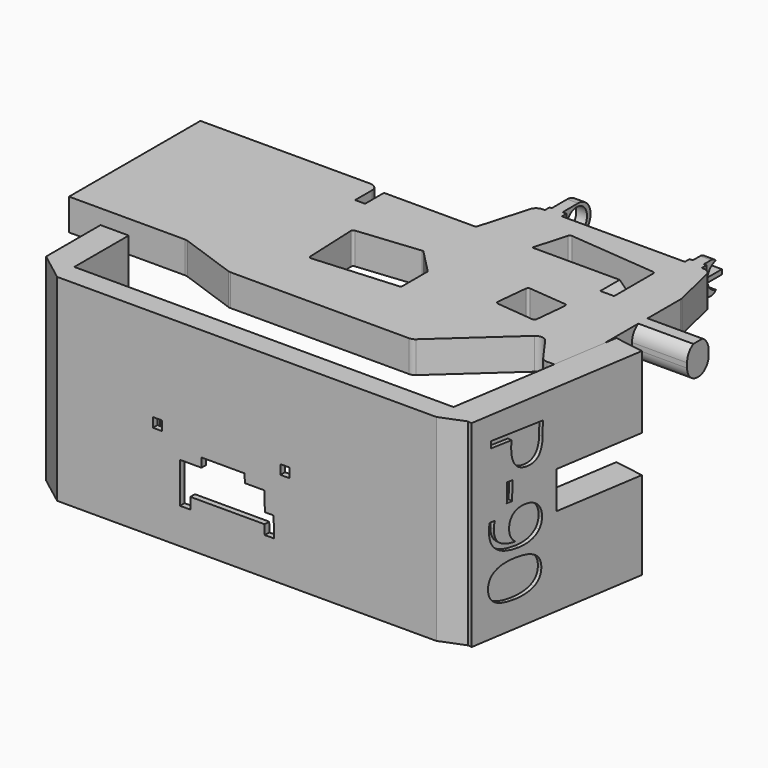
from build123d import *

# Parameters (mm, degrees)
F1_DEPTH     = 4
F3_DEPTH     = 25
F4_R         = 1.7
F5_SIZE      = 1
F7_R         = 1
F9_DEPTH     = 0.5
F10_R        = 0.2
F12_DEPTH    = 25
F13_W        = 4.2640957981
F13_H        = 4.7070300207
F13_W_2      = 7.1971410604
F14_DEPTH    = 4
F16_DEPTH    = 1.4
F17_R        = 1.99999
F18_T1_DEPTH = 5.2538537094
F19_R        = 0.3
F21_DEPTH    = 5
F22_DEPTH    = 2
F24_DEPTH    = 3
F26_DEPTH    = 0.508
F28_DEPTH    = 6.9789886475


# Not quite as in the source:
# - a fillet or chamfer that OpenCascade refuses, or shapes differently, is made with other operations: its cross-section is extruded or revolved along the edge and cut away or added
# - a fillet or chamfer is up to 0.001 mm smaller than in the source, because OpenCascade refuses the exact size


with BuildPart() as f1:
    # F0 (on Top) → F1 (new body)
    with BuildSketch(Plane.XY):
        Polygon((2.6934260968, -5.2742385305), (-19.873496145, -5.2742385305), (-19.8852140456, -26.0831601918), (-4.9857888371, -26.0831601918), (2.5662551634, -28.7642404437), (25.7749762386, -28.7642404437), (35.5768278241, -19.8526754975), (38.6626347899, -24.1568814963), (41.1353074014, -24.1568814963), (41.1353074014, -13.1260063499), (48.1142960489, -13.1260063499), (48.1142960489, -9.7081437707), (41.1497019231, -9.7081437707), (41.1497019231, -5.3435540758), (39.6437942982, 1.0947899427), (38.6000163853, 1.0947899427), (38.6000163853, 1.8441530508), (38.2520891726, 1.8441530508), (38.2520891726, 3.7778269034), (36.8706174195, 3.7778269034), (36.8706174195, 1.8408568576), (36.4612936974, 1.8441530508), (36.4612936974, 1.0947899427), (20.8624477269, 1.0947899427), (20.8624477269, 1.8441530508), (20.3708820045, 1.8408568576), (20.3410126269, 6.2953173183), (18.9800560474, 6.2953173183), (18.9800560474, 1.8365884898), (18.7107231468, 1.8365884898), (18.7107231468, 1.0847063968), (17.6446232945, 1.0847063968), (15.6181209185, -5.9725809842), (14.758749865, -8.965337649), (2.9602518771, -8.965337649), (2.6934260968, -8.965337649), align=None)
        Polygon((6.4800432883, -14.1137875617), (14.7967338562, -13.2744237781), (17.8792309016, -16.4292808622), (17.8792309016, -20.6550508738), (6.798423361, -21.4654710144), align=None, mode=Mode.SUBTRACT)
        Polygon((27.3169986904, -17.448535189), (27.7794320136, -12.9215558991), (33.1285022632, -13.4127461622), (32.6604864311, -17.9943752814), align=None, mode=Mode.SUBTRACT)
        Polygon((21.8643173575, -9.025641717), (22.7453019361, -5.9576160274), (24.017155533, -1.5283903593), (35.5836041272, -2.5712102652), (35.5836041272, -9.025641717), (34.8310694098, -9.025641717), align=None, mode=Mode.SUBTRACT)
        Polygon((2.9602518771, -5.9725809842), (2.9602518771, -8.965337649), (14.758749865, -8.965337649), (15.6181209185, -5.9725809842), align=None)
        Polygon((34.8310694098, -5.9576160274), (22.7453019361, -5.9576160274), (21.8643173575, -9.025641717), (34.8310694098, -9.025641717), align=None)
    extrude(amount=F1_DEPTH)

    # F2 (on face) → F3 (cut)
    with BuildSketch(Plane(origin=(18.9800560474, 0, 0), x_dir=(0, -1, 0), z_dir=(-1, 0, 0))):
        with BuildLine():
            ThreePointArc((-5.2999777311, 3.1070642549), (-5.723785386, 2), (-5.2999777311, 0.8929357451))
            Line((-5.2999777311, 0.8929357451), (-4.0659529041, 2))
            Line((-4.0659529041, 2), (-5.2999777311, 3.1070642549))
        make_face()
        with BuildLine():
            Line((-4.0659529041, 2), (-5.2999777311, 0.8929357451))
            ThreePointArc((-5.2999777311, 0.8929357451), (-4.0659529041, 0.342167518), (-2.831928077, 0.8929357451))
            Line((-2.831928077, 0.8929357451), (-4.0659529041, 2))
        make_face()
        with BuildLine():
            Line((-5.2999777311, 3.1070642549), (-4.0659529041, 2))
            Line((-4.0659529041, 2), (-2.831928077, 3.1070642549))
            ThreePointArc((-2.831928077, 3.1070642549), (-4.0659529041, 3.657832482), (-5.2999777311, 3.1070642549))
        make_face()
        with BuildLine():
            Line((-2.831928077, 3.1070642549), (-4.0659529041, 2))
            Line((-4.0659529041, 2), (-2.831928077, 0.8929357451))
            ThreePointArc((-2.831928077, 0.8929357451), (-2.5176934006, 1.4072934552), (-2.4081204221, 2))
            ThreePointArc((-2.4081204221, 2), (-2.5176934006, 2.5927065448), (-2.831928077, 3.1070642549))
        make_face()
    extrude(amount=-F3_DEPTH, mode=Mode.SUBTRACT)

    # F4
    f4_edges = [f1.edges().sort_by_distance(p)[0] for p in [
        (44.631999, -9.708144, 4),
        (44.631999, -9.708144, 0),
        (44.624802, -13.126006, 4),
        (44.624802, -13.126006, 0),
    ]]
    fillet(f4_edges, radius=F4_R)

    # F5
    f5_edges = [f1.edges().sort_by_distance(p)[0] for p in [
        (2.960252, -7.468959, 4),
        (2.960252, -7.468959, 0),
        (34.831069, -7.491629, 4),
        (34.831069, -7.491629, 0),
    ]]
    chamfer(f5_edges, length=F5_SIZE)

    # F7
    f7_edges = [f1.edges().sort_by_distance(p)[0] for p in [
        (-4.985789, -26.08316, 2),
        (2.566255, -28.76424, 2),
        (25.774976, -28.76424, 2),
        (35.576828, -19.852675, 2),
        (38.662635, -24.156881, 2),
        (41.135307, -24.156881, 2),
        (41.149702, -5.343554, 2),
        (39.643794, 1.09479, 2),
        (17.644623, 1.084706, 2),
        (2.693426, -5.274239, 2),
    ]]
    fillet(f7_edges, radius=F7_R)

    # F8 (on face) → F9 (join)
    with BuildSketch(Plane(origin=(0, -5.9725809842, 0), x_dir=(-1, 0, 0), z_dir=(0, 1, 0))):
        Polygon((-4.663484171, 0.6533203996), (-4.2501688004, 0.6387769245), (-4.2501688004, 3.2442298252), (-4.663484171, 3.2442298252), align=None)
        Polygon((-7, 0.6), (-6.5866846293, 0.5854565249), (-6.5866846293, 3.1909094256), (-7, 3.1909094256), align=None)
        Polygon((-9.336515829, 0.5466796004), (-8.9232004583, 0.5321361253), (-8.9232004583, 3.1375890261), (-9.336515829, 3.1375890261), align=None)
        Polygon((-11.6730316579, 0.4933592008), (-11.2597162873, 0.4788157257), (-11.2597162873, 3.0842686265), (-11.6730316579, 3.0842686265), align=None)
        Polygon((-14.0095474869, 0.4400388013), (-13.5962321162, 0.4254953261), (-13.5962321162, 3.0309482269), (-14.0095474869, 3.0309482269), align=None)
        Polygon((-16.3460633159, 0.3867184017), (-15.9327479452, 0.3721749266), (-15.9327479452, 2.9776278273), (-16.3460633159, 2.9776278273), align=None)
        Polygon((-18.6825791448, 0.3333980021), (-18.2692637742, 0.318854527), (-18.2692637742, 2.9243074277), (-18.6825791448, 2.9243074277), align=None)
        Polygon((-21.0190949738, 0.2800776025), (-20.6057796031, 0.2655341274), (-20.6057796031, 2.8709870282), (-21.0190949738, 2.8709870282), align=None)
        Polygon((-23.3556108028, 0.2267572029), (-22.9422954321, 0.2122137278), (-22.9422954321, 2.8176666286), (-23.3556108028, 2.8176666286), align=None)
        Polygon((-25.6921266317, 0.1734368034), (-25.2788112611, 0.1588933283), (-25.2788112611, 2.764346229), (-25.6921266317, 2.764346229), align=None)
        Polygon((-28.0286424607, 0.1201164038), (-27.61532709, 0.1055729287), (-27.61532709, 2.7110258294), (-28.0286424607, 2.7110258294), align=None)
        Polygon((-30.3651582897, 0.0667960042), (-29.951842919, 0.0522525291), (-29.951842919, 2.6577054298), (-30.3651582897, 2.6577054298), align=None)
        Polygon((-32.7016741186, 0.0134756046), (-32.288358748, -0.0010678705), (-32.288358748, 2.6043850303), (-32.7016741186, 2.6043850303), align=None)
    extrude(amount=F9_DEPTH)

    # F10
    f10_edges = [f1.edges().sort_by_distance(p)[0] for p in [
        (4.250169, -5.472581, 1.941503),
        (4.663484, -5.472581, 1.948775),
        (6.586685, -5.472581, 1.888183),
        (7, -5.472581, 1.895455),
        (8.9232, -5.472581, 1.834863),
        (9.336516, -5.472581, 1.842134),
        (11.259716, -5.472581, 1.781542),
        (11.673032, -5.472581, 1.788814),
        (13.596232, -5.472581, 1.728222),
        (14.009547, -5.472581, 1.735494),
        (23.355611, -5.472581, 1.522212),
        (22.942295, -5.472581, 1.51494),
        (25.692127, -5.472581, 1.468892),
        (25.278811, -5.472581, 1.46162),
        (27.615327, -5.472581, 1.408299),
        (28.028642, -5.472581, 1.415571),
        (29.951843, -5.472581, 1.354979),
        (30.365158, -5.472581, 1.362251),
        (32.288359, -5.472581, 1.301659),
        (32.701674, -5.472581, 1.30893),
    ]]
    fillet(f10_edges, radius=F10_R)

    # F15 (on face) → F16 (join)
    with BuildSketch(Plane(origin=(36.8706174195, 0, 0), x_dir=(0, -1, 0), z_dir=(-1, 0, 0))):
        with BuildLine():
            ThreePointArc((-2.4346986369, 1.7043345571), (-2.414778345, 1.8515711823), (-2.4081204221, 2))
            Line((-2.4081204221, 2), (-4.7012325376, 2))
            Line((-4.7012325376, 2), (-4.7012325376, 1.7043345571))
            Line((-4.7012325376, 1.7043345571), (-2.4346986369, 1.7043345571))
        make_face()
        with BuildLine():
            Line((-4.7012325376, 2), (-2.4081204221, 2))
            ThreePointArc((-2.4081204221, 2), (-2.414778345, 2.1484288177), (-2.4346986369, 2.2956654429))
            Line((-2.4346986369, 2.2956654429), (-4.7012325376, 2.2956654429))
            Line((-4.7012325376, 2.2956654429), (-4.7012325376, 2))
        make_face()
    extrude(amount=-F16_DEPTH)

    # F17 (radius 2 in the source; OpenCascade refuses exactly that, so slightly less here)
    f17_edges = [f1.edges().sort_by_distance(p)[0] for p in [
        (19.660534, 6.295317, 0),
        (19.660534, 6.295317, 4),
    ]]
    fillet(f17_edges, radius=F17_R)

    # F18: fillet of radius 1 on 2 edges, made by hand

    # F18_s2 → F18_t1 (cut)
    with BuildSketch(Plane.YZ.offset(34.9344264413)):
        with BuildLine():
            ThreePointArc((3.0033505121, 4), (3.431951251, 3.9034939992), (3.7778269034, 3.6326028133))
            Line((3.7778269034, 3.6326028133), (3.7778269034, 4))
            Line((3.7778269034, 4), (3.0033505121, 4))
        make_face()
        with BuildLine():
            ThreePointArc((3.0033505121, 0), (3.431951251, 0.0965060008), (3.7778269034, 0.3673971867))
            Line((3.7778269034, 0.3673971867), (3.7778269034, 0))
            Line((3.7778269034, 0), (3.0033505121, 0))
        make_face()
    extrude(amount=F18_T1_DEPTH, mode=Mode.SUBTRACT)

    # F19
    f19_edges = [f1.edges().sort_by_distance(p)[0] for p in [
        (24.017156, -1.52839, 2),
        (35.583604, -2.57121, 2),
        (33.128502, -13.412746, 2),
        (32.660486, -17.994375, 2),
        (27.316999, -17.448535, 2),
        (27.779432, -12.921556, 2),
        (17.879231, -16.429281, 2),
        (17.879231, -20.655051, 2),
        (14.796734, -13.274424, 2),
        (6.480043, -14.113788, 2),
        (6.798423, -21.465471, 2),
    ]]
    fillet(f19_edges, radius=F19_R)

    # F27 (on face) → F28 (join, through all)
    with BuildSketch(Plane.YZ.offset(48.1142960489)):
        with BuildLine():
            Line((-9.7081437707, 2.3), (-13.1260063499, 2.3))
            Line((-13.1260063499, 2.3), (-13.1260063499, 1.7))
            ThreePointArc((-13.1260063499, 1.7), (-12.6280878779, 0.497918472), (-11.4260063499, 0))
            Line((-11.4260063499, 0), (-11.4081437707, 0))
            ThreePointArc((-11.4081437707, 0), (-10.2060622427, 0.497918472), (-9.7081437707, 1.7))
            Line((-9.7081437707, 1.7), (-9.7081437707, 2.3))
        make_face()
        with BuildLine():
            Line((-11.4081437707, 4), (-11.4260063499, 4))
            ThreePointArc((-11.4260063499, 4), (-12.6280878779, 3.502081528), (-13.1260063499, 2.3))
            Line((-13.1260063499, 2.3), (-9.7081437707, 2.3))
            ThreePointArc((-9.7081437707, 2.3), (-10.2060622427, 3.502081528), (-11.4081437707, 4))
        make_face()
        with BuildLine():
            ThreePointArc((-13.1260063499, 2.3), (-12.6280878779, 3.502081528), (-11.4260063499, 4))
            Line((-11.4260063499, 4), (-12.1334744617, 4))
            ThreePointArc((-12.1334744617, 4), (-12.8597103306, 3.2842661669), (-13.1260063499, 2.3))
        make_face()
        with BuildLine():
            Line((-10.6828130797, 4), (-11.4081437707, 4))
            ThreePointArc((-11.4081437707, 4), (-10.2060622427, 3.502081528), (-9.7081437707, 2.3))
            ThreePointArc((-9.7081437707, 2.3), (-9.9667172587, 3.2811567577), (-10.6828130797, 4))
        make_face()
    extrude(amount=-F28_DEPTH)


with BuildPart() as f12:
    # F11 (on face) → F12 (new body)
    with BuildSketch(Plane.XY.offset(4)):
        Polygon((44.5833335705, -16.4324613858), (41.3761623204, -15.9014053643), (38.0217470229, -37.5300385058), (-10.0583480671, -37.5300385058), (-10.0583480671, -28.9046149701), (-13.636412099, -28.9046149701), (-13.636412099, -37.5300385058), (-10.0583480671, -40.2552820742), (38.0217470229, -40.2552820742), (41.0766750574, -39.0427298844), align=None)
    extrude(amount=-F12_DEPTH)

    # F13 (on face) → F14 (cut)
    with BuildSketch(Plane(origin=(46.0248163774, -7.1380538526, 0), x_dir=(0.1532591685, 0.9881860287, 0), z_dir=(0.9881860287, -0.1532591685, 0))):
        Polygon((-7.2025824338, -5.1408624277), (-9.4055241255, -5.1408624277), (-16.6026651859, -5.1408624277), (-16.6026651859, -9.8478924483), (-9.4055241255, -9.8478924483), (-7.2025824338, -10.2310068905), align=None)
        with Locations((-18.734713085, -7.494377438)):
            Rectangle(F13_W, F13_H)
        with Locations((-13.0040946557, -7.494377438)):
            Rectangle(F13_W_2, F13_H)
    extrude(amount=-F14_DEPTH, mode=Mode.SUBTRACT)

    # F20 (on face) → F21 (cut)
    with BuildSketch(Plane(origin=(0, -37.5300385058, 0), x_dir=(-1, 0, 0), z_dir=(0, 1, 0))):
        Polygon((-10.7441206637, -15.0589602471), (-10.7441206637, -10.204165907), (-13.7182893232, -10.204165907), (-13.74556683, -11.2833930179), (-16.2131562829, -11.2833930179), (-16.2884704769, -13.7014463544), (-17.4019206315, -13.7014463544), (-17.4291040748, -16.2507686764), (-16.2706725371, -16.2631210407), (-16.2578325614, -15.0589602471), align=None)
        Polygon((-8.2328791401, -10.204165907), (-10.7441206637, -10.204165907), (-10.7441206637, -15.0589602471), (-6.8352012895, -15.0589602471), (-6.8352012895, -16.4881702513), (-5.5278930813, -16.4881702513), (-5.5278930813, -11.3542200997), (-8.2451421767, -11.3542200997), align=None)
        Polygon((-18.2534381747, -7.6958201826), (-19.4096304476, -7.6958201826), (-19.4027870893, -8.8917091489), (-18.2534381747, -8.8917091489), align=None)
        Polygon((-2.0786108798, -7.6958201826), (-3.2348031527, -7.6958201826), (-3.2348031527, -8.8917091489), (-2.0854542381, -8.8917091489), align=None)
    extrude(amount=-F21_DEPTH, mode=Mode.SUBTRACT)

    # F20 (on face) → F22 (cut)
    with BuildSketch(Plane(origin=(0, -37.5300385058, 0), x_dir=(-1, 0, 0), z_dir=(0, 1, 0))):
        Polygon((-0.7839830942, 1.2256489135), (-10.7441206637, 1.2256489135), (-10.7441206637, -10.204165907), (-8.2328791401, -10.204165907), (-8.2451421767, -11.3542200997), (-5.5278930813, -11.3542200997), (-5.5278930813, -16.4881702513), (-6.8352012895, -16.4881702513), (-6.8352012895, -15.0589602471), (-10.7441206637, -15.0589602471), (-10.7441206637, -18.6946262256), (-0.7839830942, -18.6946262256), align=None)
        Polygon((-3.2348031527, -8.8917091489), (-3.2348031527, -7.6958201826), (-2.0786108798, -7.6958201826), (-2.0854542381, -8.8917091489), align=None, mode=Mode.SUBTRACT)
        Polygon((-10.7441206637, 1.2256489135), (-20.7042582333, 1.2256489135), (-20.7042582333, -18.6946262256), (-10.7441206637, -18.6946262256), (-10.7441206637, -15.0589602471), (-16.2578325614, -15.0589602471), (-16.2706725371, -16.2631210407), (-17.4291040748, -16.2507686764), (-17.4019206315, -13.7014463544), (-16.2884704769, -13.7014463544), (-16.2131562829, -11.2833930179), (-13.74556683, -11.2833930179), (-13.7182893232, -10.204165907), (-10.7441206637, -10.204165907), align=None)
        Polygon((-19.4027870893, -8.8917091489), (-19.4096304476, -7.6958201826), (-18.2534381747, -7.6958201826), (-18.2534381747, -8.8917091489), align=None, mode=Mode.SUBTRACT)
    extrude(amount=-F22_DEPTH, mode=Mode.SUBTRACT)

    # F23 (on face) → F24 (cut)
    with BuildSketch(Plane(origin=(-13.636412099, 0, 0), x_dir=(0, -1, 0), z_dir=(-1, 0, 0))):
        with BuildLine():
            Line((35.6485965423, -20.3161685267), (33.5925474496, -20.1962334233))
            Line((33.5925474496, -20.1962334233), (33.6680283577, -20.6826224671))
            Line((33.6680283577, -20.6826224671), (35.6674124532, -20.800094644))
            add(Edge.make_bspline(
                [(36.170021659, -20.7868217916), (35.9923202004, -20.8143986206), (35.6674124532, -20.800094644)],
                knots=[0, 0, 0, 1, 1, 1], degree=2))
            add(Edge.make_bspline(
                [(36.7059816488, -20.4897735703), (36.5391643796, -20.7295359047), (36.170021659, -20.7868217916)],
                knots=[0, 0, 0, 1, 1, 1], degree=2))
            add(Edge.make_bspline(
                [(36.8159394769, -19.8836164761), (36.8727989181, -20.250011236), (36.7059816488, -20.4897735703)],
                knots=[0, 0, 0, 1, 1, 1], degree=2))
            add(Edge.make_bspline(
                [(36.5935289668, -19.3782858258), (36.7737213418, -19.6115683668), (36.8159394769, -19.8836164761)],
                knots=[0, 0, 0, 1, 1, 1], degree=2))
            add(Edge.make_bspline(
                [(36.0126042282, -18.9201492485), (36.4133365917, -19.1450032847), (36.5935289668, -19.3782858258)],
                knots=[0, 0, 0, 1, 1, 1], degree=2))
            Line((36.0126042282, -18.9201492485), (36.0073447299, -18.8862577332))
            Line((36.0073447299, -18.8862577332), (36.5977465295, -18.8584226281))
            Line((36.5977465295, -18.8584226281), (36.5360540358, -18.4608843136))
            Line((36.5360540358, -18.4608843136), (33.2961676124, -18.286400737))
            Line((33.2961676124, -18.286400737), (33.3699427373, -18.7617979381))
            Line((33.3699427373, -18.7617979381), (34.7736176608, -18.836637324))
            add(Edge.make_bspline(
                [(35.5907766713, -19.0006198421), (35.2413250899, -18.8644265124), (34.7736176608, -18.836637324)],
                knots=[0, 0, 0, 1, 1, 1], degree=2))
            add(Edge.make_bspline(
                [(36.1497162504, -19.3533548306), (35.9402282526, -19.1368131717), (35.5907766713, -19.0006198421)],
                knots=[0, 0, 0, 1, 1, 1], degree=2))
            add(Edge.make_bspline(
                [(36.3982951141, -19.8217928869), (36.3592042482, -19.5698964894), (36.1497162504, -19.3533548306)],
                knots=[0, 0, 0, 1, 1, 1], degree=2))
            add(Edge.make_bspline(
                [(36.0542373272, -20.3066872863), (36.4636834714, -20.2431468608), (36.3982951141, -19.8217928869)],
                knots=[0, 0, 0, 1, 1, 1], degree=2))
            add(Edge.make_bspline(
                [(35.6485965423, -20.3161685267), (35.9113433708, -20.3288624684), (36.0542373272, -20.3066872863)],
                knots=[0, 0, 0, 1, 1, 1], degree=2))
        make_face()
        with BuildLine():
            Line((34.0340840387, -15.4130917276), (36.0811785063, -15.529726234))
            Line((36.0811785063, -15.529726234), (36.0056975981, -15.0433371902))
            Line((36.0056975981, -15.0433371902), (34.0185846828, -14.9324031122))
            add(Edge.make_bspline(
                [(33.4926493588, -14.9464817188), (33.7188981231, -14.9113710139), (34.0185846828, -14.9324031122)],
                knots=[0, 0, 0, 1, 1, 1], degree=2))
            add(Edge.make_bspline(
                [(32.9688104215, -15.2430559887), (33.1354144678, -15.001919674), (33.4926493588, -14.9464817188)],
                knots=[0, 0, 0, 1, 1, 1], degree=2))
            add(Edge.make_bspline(
                [(32.8586393705, -15.8478391026), (32.8022063752, -15.4841923033), (32.9688104215, -15.2430559887)],
                knots=[0, 0, 0, 1, 1, 1], degree=2))
            add(Edge.make_bspline(
                [(33.0857404161, -16.3561940318), (32.9012839514, -16.1226351725), (32.8586393705, -15.8478391026)],
                knots=[0, 0, 0, 1, 1, 1], degree=2))
            add(Edge.make_bspline(
                [(33.6618324706, -16.8103903433), (33.2701968808, -16.589752891), (33.0857404161, -16.3561940318)],
                knots=[0, 0, 0, 1, 1, 1], degree=2))
            Line((33.6618324706, -16.8103903433), (33.6663812259, -16.839701924))
            Line((33.6663812259, -16.839701924), (33.0758372778, -16.8666210422))
            Line((33.0758372778, -16.8666210422), (33.1375297715, -17.2641593568))
            Line((33.1375297715, -17.2641593568), (36.3788376809, -17.4478028023))
            Line((36.3788376809, -17.4478028023), (36.3042096643, -16.9669096799))
            Line((36.3042096643, -16.9669096799), (34.8999661464, -16.8884063463))
            add(Edge.make_bspline(
                [(34.086336914, -16.7290353104), (34.4328273117, -16.8642811055), (34.8999661464, -16.8884063463)],
                knots=[0, 0, 0, 1, 1, 1], degree=2))
            add(Edge.make_bspline(
                [(33.5305717413, -16.3786218368), (33.7398465162, -16.5937895153), (34.086336914, -16.7290353104)],
                knots=[0, 0, 0, 1, 1, 1], degree=2))
            add(Edge.make_bspline(
                [(33.2816375062, -15.9078938132), (33.3212969664, -16.1634541583), (33.5305717413, -16.3786218368)],
                knots=[0, 0, 0, 1, 1, 1], degree=2))
            add(Edge.make_bspline(
                [(33.3403193418, -15.5667187669), (33.2470953957, -15.6853089966), (33.2816375062, -15.9078938132)],
                knots=[0, 0, 0, 1, 1, 1], degree=2))
            add(Edge.make_bspline(
                [(33.6130767203, -15.4202674111), (33.433543288, -15.4481285373), (33.3403193418, -15.5667187669)],
                knots=[0, 0, 0, 1, 1, 1], degree=2))
            add(Edge.make_bspline(
                [(34.0340840387, -15.4130917276), (33.7275750828, -15.4024988357), (33.6130767203, -15.4202674111)],
                knots=[0, 0, 0, 1, 1, 1], degree=2))
        make_face()
        with BuildLine():
            add(Edge.make_bspline(
                [(35.369233503, -13.154387338), (35.3447839433, -12.9968375912), (35.2310716928, -12.7537072699)],
                knots=[0, 0, 0, 1, 1, 1], degree=2))
            add(Edge.make_bspline(
                [(35.3194812501, -13.3989649246), (35.3922615767, -13.3027772158), (35.369233503, -13.154387338)],
                knots=[0, 0, 0, 1, 1, 1], degree=2))
            add(Edge.make_bspline(
                [(35.0864032161, -13.520028639), (35.2467009236, -13.4951526334), (35.3194812501, -13.3989649246)],
                knots=[0, 0, 0, 1, 1, 1], degree=2))
            add(Edge.make_bspline(
                [(34.7001403047, -13.5274407456), (34.9572490632, -13.540071592), (35.0864032161, -13.520028639)],
                knots=[0, 0, 0, 1, 1, 1], degree=2))
            Line((34.7001403047, -13.5274407456), (32.9143871376, -13.4265324387))
            Line((32.9143871376, -13.4265324387), (32.7931343793, -12.6451956132))
            Line((32.7931343793, -12.6451956132), (32.4179735432, -12.6274336696))
            Line((32.4179735432, -12.6274336696), (32.5396527474, -13.4115184559))
            Line((32.5396527474, -13.4115184559), (31.7934055106, -13.3659818083))
            Line((31.7934055106, -13.3659818083), (31.8369029831, -13.6462737997))
            Line((31.8369029831, -13.6462737997), (32.5455817464, -13.9030727236))
            Line((32.5455817464, -13.9030727236), (32.8512444425, -14.3978288926))
            Line((32.8512444425, -14.3978288926), (33.0663439942, -14.4057224347))
            Line((33.0663439942, -14.4057224347), (32.9898680458, -13.9129214826))
            Line((32.9898680458, -13.9129214826), (34.7692723998, -14.0091867596))
            add(Edge.make_bspline(
                [(35.2068305777, -13.9938143312), (35.0181372763, -14.0230969434), (34.7692723998, -14.0091867596)],
                knots=[0, 0, 0, 1, 1, 1], degree=2))
            add(Edge.make_bspline(
                [(35.685707472, -13.7248545749), (35.5448297437, -13.9413614967), (35.2068305777, -13.9938143312)],
                knots=[0, 0, 0, 1, 1, 1], degree=2))
            add(Edge.make_bspline(
                [(35.7710050965, -13.1501967751), (35.8265852002, -13.508347653), (35.685707472, -13.7248545749)],
                knots=[0, 0, 0, 1, 1, 1], degree=2))
            add(Edge.make_bspline(
                [(35.7066143584, -12.9256777312), (35.7576431278, -13.0640940066), (35.7710050965, -13.1501967751)],
                knots=[0, 0, 0, 1, 1, 1], degree=2))
            add(Edge.make_bspline(
                [(35.6002144135, -12.6964213829), (35.655585589, -12.7872614558), (35.7066143584, -12.9256777312)],
                knots=[0, 0, 0, 1, 1, 1], degree=2))
            Line((35.6002144135, -12.6964213829), (35.2310716928, -12.7537072699))
        make_face()
        with BuildLine():
            Line((34.3034443124, -11.6481844933), (32.2473952196, -11.5282493898))
            Line((32.2473952196, -11.5282493898), (32.3228761278, -12.0146384336))
            Line((32.3228761278, -12.0146384336), (34.3222602233, -12.1321106105))
            add(Edge.make_bspline(
                [(34.824869429, -12.1188377582), (34.6471679705, -12.1464145872), (34.3222602233, -12.1321106105)],
                knots=[0, 0, 0, 1, 1, 1], degree=2))
            add(Edge.make_bspline(
                [(35.3608294189, -11.8217895369), (35.1940121497, -12.0615518712), (34.824869429, -12.1188377582)],
                knots=[0, 0, 0, 1, 1, 1], degree=2))
            add(Edge.make_bspline(
                [(35.470787247, -11.2156324426), (35.5276466882, -11.5820272026), (35.3608294189, -11.8217895369)],
                knots=[0, 0, 0, 1, 1, 1], degree=2))
            add(Edge.make_bspline(
                [(35.2483767368, -10.7103017923), (35.4285691119, -10.9435843334), (35.470787247, -11.2156324426)],
                knots=[0, 0, 0, 1, 1, 1], degree=2))
            add(Edge.make_bspline(
                [(34.6674519983, -10.252165215), (35.0681843618, -10.4770192512), (35.2483767368, -10.7103017923)],
                knots=[0, 0, 0, 1, 1, 1], degree=2))
            Line((34.6674519983, -10.252165215), (34.6621925, -10.2182736997))
            Line((34.6621925, -10.2182736997), (35.2525942995, -10.1904385947))
            Line((35.2525942995, -10.1904385947), (35.1909018058, -9.7929002801))
            Line((35.1909018058, -9.7929002801), (31.9510153825, -9.6184167036))
            Line((31.9510153825, -9.6184167036), (32.0247905074, -10.0938139046))
            Line((32.0247905074, -10.0938139046), (33.4284654309, -10.1686532906))
            add(Edge.make_bspline(
                [(34.2456244413, -10.3326358086), (33.89617286, -10.196442479), (33.4284654309, -10.1686532906)],
                knots=[0, 0, 0, 1, 1, 1], degree=2))
            add(Edge.make_bspline(
                [(34.8045640205, -10.6853707971), (34.5950760227, -10.4688291382), (34.2456244413, -10.3326358086)],
                knots=[0, 0, 0, 1, 1, 1], degree=2))
            add(Edge.make_bspline(
                [(35.0531428841, -11.1538088534), (35.0140520183, -10.901912456), (34.8045640205, -10.6853707971)],
                knots=[0, 0, 0, 1, 1, 1], degree=2))
            add(Edge.make_bspline(
                [(34.7090850973, -11.6387032529), (35.1185312415, -11.5751628274), (35.0531428841, -11.1538088534)],
                knots=[0, 0, 0, 1, 1, 1], degree=2))
            add(Edge.make_bspline(
                [(34.3034443124, -11.6481844933), (34.5661911409, -11.660878435), (34.7090850973, -11.6387032529)],
                knots=[0, 0, 0, 1, 1, 1], degree=2))
        make_face()
        with BuildLine():
            add(Edge.make_bspline(
                [(31.5308292702, -7.2916054709), (31.5001251719, -7.0937523005), (31.5178269677, -6.9418558449)],
                knots=[0, 0, 0, 1, 1, 1], degree=2))
            add(Edge.make_bspline(
                [(31.6462955465, -7.6095073045), (31.558832545, -7.4720548902), (31.5308292702, -7.2916054709)],
                knots=[0, 0, 0, 1, 1, 1], degree=2))
            add(Edge.make_bspline(
                [(31.8732036219, -7.8627435557), (31.733758548, -7.7469597189), (31.6462955465, -7.6095073045)],
                knots=[0, 0, 0, 1, 1, 1], degree=2))
            add(Edge.make_bspline(
                [(32.3166802407, -8.1424063098), (32.0126486957, -7.9785273924), (31.8732036219, -7.8627435557)],
                knots=[0, 0, 0, 1, 1, 1], degree=2))
            Line((32.3166802407, -8.1424063098), (32.321228996, -8.1717178906))
            Line((32.321228996, -8.1717178906), (31.7306850479, -8.1986370088))
            Line((31.7306850479, -8.1986370088), (31.7923775415, -8.5961753233))
            Line((31.7923775415, -8.5961753233), (35.033685451, -8.7798187689))
            Line((35.033685451, -8.7798187689), (34.9590574344, -8.2989256464))
            Line((34.9590574344, -8.2989256464), (33.4742542065, -8.215101193))
            add(Edge.make_bspline(
                [(32.7585333189, -8.070084587), (33.0899965967, -8.1931226655), (33.4742542065, -8.215101193)],
                knots=[0, 0, 0, 1, 1, 1], degree=2))
            add(Edge.make_bspline(
                [(32.2199985695, -7.7460766268), (32.4270700411, -7.9470465084), (32.7585333189, -8.070084587)],
                knots=[0, 0, 0, 1, 1, 1], degree=2))
            add(Edge.make_bspline(
                [(31.9725568947, -7.2849664657), (32.012927098, -7.5451067453), (32.2199985695, -7.7460766268)],
                knots=[0, 0, 0, 1, 1, 1], degree=2))
            add(Edge.make_bspline(
                [(31.9633454672, -6.9777786829), (31.9493866724, -7.135660601), (31.9725568947, -7.2849664657)],
                knots=[0, 0, 0, 1, 1, 1], degree=2))
            Line((31.9633454672, -6.9777786829), (31.5178269677, -6.9418558449))
        make_face()
        with BuildLine():
            Line((32.3287272488, -4.4239968899), (34.3758217164, -4.5406313963))
            Line((34.3758217164, -4.5406313963), (34.3003408082, -4.0542423524))
            Line((34.3003408082, -4.0542423524), (32.313227893, -3.9433082744))
            add(Edge.make_bspline(
                [(31.7872925689, -3.9573868811), (32.0135413332, -3.9222761762), (32.313227893, -3.9433082744)],
                knots=[0, 0, 0, 1, 1, 1], degree=2))
            add(Edge.make_bspline(
                [(31.2634536317, -4.2539611509), (31.430057678, -4.0128248363), (31.7872925689, -3.9573868811)],
                knots=[0, 0, 0, 1, 1, 1], degree=2))
            add(Edge.make_bspline(
                [(31.1532825807, -4.8587442649), (31.0968495853, -4.4950974656), (31.2634536317, -4.2539611509)],
                knots=[0, 0, 0, 1, 1, 1], degree=2))
            add(Edge.make_bspline(
                [(31.3803836263, -5.3670991941), (31.1959271616, -5.1335403348), (31.1532825807, -4.8587442649)],
                knots=[0, 0, 0, 1, 1, 1], degree=2))
            add(Edge.make_bspline(
                [(31.9564756807, -5.8212955055), (31.564840091, -5.6006580533), (31.3803836263, -5.3670991941)],
                knots=[0, 0, 0, 1, 1, 1], degree=2))
            Line((31.9564756807, -5.8212955055), (31.961024436, -5.8506070863))
            Line((31.961024436, -5.8506070863), (31.3704804879, -5.8775262045))
            Line((31.3704804879, -5.8775262045), (31.4321729816, -6.2750645191))
            Line((31.4321729816, -6.2750645191), (34.673480891, -6.4587079646))
            Line((34.673480891, -6.4587079646), (34.5988528745, -5.9778148422))
            Line((34.5988528745, -5.9778148422), (33.1946093565, -5.8993115086))
            add(Edge.make_bspline(
                [(32.3809801241, -5.7399404727), (32.7274705219, -5.8751862678), (33.1946093565, -5.8993115086)],
                knots=[0, 0, 0, 1, 1, 1], degree=2))
            add(Edge.make_bspline(
                [(31.8252149515, -5.3895269991), (32.0344897264, -5.6046946776), (32.3809801241, -5.7399404727)],
                knots=[0, 0, 0, 1, 1, 1], degree=2))
            add(Edge.make_bspline(
                [(31.5762807163, -4.9187989755), (31.6159401766, -5.1743593206), (31.8252149515, -5.3895269991)],
                knots=[0, 0, 0, 1, 1, 1], degree=2))
            add(Edge.make_bspline(
                [(31.634962552, -4.5776239292), (31.5417386058, -4.6962141589), (31.5762807163, -4.9187989755)],
                knots=[0, 0, 0, 1, 1, 1], degree=2))
            add(Edge.make_bspline(
                [(31.9077199305, -4.4311725734), (31.7281864981, -4.4590336996), (31.634962552, -4.5776239292)],
                knots=[0, 0, 0, 1, 1, 1], degree=2))
            add(Edge.make_bspline(
                [(32.3287272488, -4.4239968899), (32.022218293, -4.413403998), (31.9077199305, -4.4311725734)],
                knots=[0, 0, 0, 1, 1, 1], degree=2))
        make_face()
        with BuildLine():
            add(Edge.make_bspline(
                [(34.0136219179, -1.8258507321), (34.0953573646, -2.3525431995), (33.8297016479, -2.7019175697)],
                knots=[0, 0, 0, 1, 1, 1], degree=2))
            add(Edge.make_bspline(
                [(33.8927369314, -1.3793394029), (33.9750996465, -1.5776182822), (34.0136219179, -1.8258507321)],
                knots=[0, 0, 0, 1, 1, 1], degree=2))
            add(Edge.make_bspline(
                [(33.6430923216, -0.9312347336), (33.8103742162, -1.1810605236), (33.8927369314, -1.3793394029)],
                knots=[0, 0, 0, 1, 1, 1], degree=2))
            Line((33.6430923216, -0.9312347336), (33.2244863084, -0.9961966452))
            add(Edge.make_bspline(
                [(33.487128431, -1.4404081859), (33.4058082617, -1.2579143068), (33.2244863084, -0.9961966452)],
                knots=[0, 0, 0, 1, 1, 1], degree=2))
            add(Edge.make_bspline(
                [(33.596451875, -1.8033514843), (33.5684486002, -1.622902065), (33.487128431, -1.4404081859)],
                knots=[0, 0, 0, 1, 1, 1], degree=2))
            add(Edge.make_bspline(
                [(33.4703533068, -2.3810578684), (33.653737762, -2.1724942049), (33.596451875, -1.8033514843)],
                knots=[0, 0, 0, 1, 1, 1], degree=2))
            add(Edge.make_bspline(
                [(32.9123302096, -2.6477603105), (33.2869688516, -2.5896215319), (33.4703533068, -2.3810578684)],
                knots=[0, 0, 0, 1, 1, 1], degree=2))
            Line((32.9123302096, -2.6477603105), (32.6816277014, -2.6723056184))
            Line((32.6816277014, -2.6723056184), (32.6669863953, -2.5779589677))
            add(Edge.make_bspline(
                [(32.1623219184, -1.2632770487), (32.5296708448, -1.6931156225), (32.6669863953, -2.5779589677)],
                knots=[0, 0, 0, 1, 1, 1], degree=2))
            add(Edge.make_bspline(
                [(31.2801883544, -0.9133259898), (31.7949729921, -0.8334384749), (32.1623219184, -1.2632770487)],
                knots=[0, 0, 0, 1, 1, 1], degree=2))
            add(Edge.make_bspline(
                [(30.7831737658, -1.2165250224), (30.9394412276, -0.9662052701), (31.2801883544, -0.9133259898)],
                knots=[0, 0, 0, 1, 1, 1], degree=2))
            add(Edge.make_bspline(
                [(30.6948533361, -1.9046865128), (30.6269063039, -1.4668447746), (30.7831737658, -1.2165250224)],
                knots=[0, 0, 0, 1, 1, 1], degree=2))
            add(Edge.make_bspline(
                [(31.0899781985, -2.6374248426), (30.7605259907, -2.3278724605), (30.6948533361, -1.9046865128)],
                knots=[0, 0, 0, 1, 1, 1], degree=2))
            add(Edge.make_bspline(
                [(31.9467259633, -3.0837130011), (31.4194304063, -2.9469772247), (31.0899781985, -2.6374248426)],
                knots=[0, 0, 0, 1, 1, 1], degree=2))
            add(Edge.make_bspline(
                [(33.0117058305, -3.1370075475), (32.4740215202, -3.2204487775), (31.9467259633, -3.0837130011)],
                knots=[0, 0, 0, 1, 1, 1], degree=2))
            add(Edge.make_bspline(
                [(33.8297016479, -2.7019175697), (33.5640459311, -3.0512919399), (33.0117058305, -3.1370075475)],
                knots=[0, 0, 0, 1, 1, 1], degree=2))
        make_face()
        with BuildLine():
            add(Edge.make_bspline(
                [(31.108706087, -1.8695416811), (31.1544779372, -2.1644894629), (31.4640061404, -2.3819220663)],
                knots=[0, 0, 0, 1, 1, 1], degree=2))
            add(Edge.make_bspline(
                [(31.1581174527, -1.526053099), (31.0740218279, -1.6460408776), (31.108706087, -1.8695416811)],
                knots=[0, 0, 0, 1, 1, 1], degree=2))
            add(Edge.make_bspline(
                [(31.3942669029, -1.3824686523), (31.2422130775, -1.4060653204), (31.1581174527, -1.526053099)],
                knots=[0, 0, 0, 1, 1, 1], degree=2))
            add(Edge.make_bspline(
                [(31.9420003111, -1.6539255772), (31.7176102785, -1.3322901954), (31.3942669029, -1.3824686523)],
                knots=[0, 0, 0, 1, 1, 1], degree=2))
            add(Edge.make_bspline(
                [(32.2676001489, -2.6277436317), (32.1663903436, -1.975560959), (31.9420003111, -1.6539255772)],
                knots=[0, 0, 0, 1, 1, 1], degree=2))
            Line((32.2676001489, -2.6277436317), (32.2730017958, -2.6625511339))
            add(Edge.make_bspline(
                [(31.4640061404, -2.3819220663), (31.7735343436, -2.5993546697), (32.2730017958, -2.6625511339)],
                knots=[0, 0, 0, 1, 1, 1], degree=2))
        make_face(mode=Mode.SUBTRACT)
        with BuildLine():
            add(Edge.make_bspline(
                [(30.2534971451, 0.981667262), (30.1673550917, 1.5367553234), (30.6718709033, 1.8701978817)],
                knots=[0, 0, 0, 1, 1, 1], degree=2))
            add(Edge.make_bspline(
                [(30.6530046771, 0.2388215286), (30.3210177315, 0.5465734846), (30.2534971451, 0.981667262)],
                knots=[0, 0, 0, 1, 1, 1], degree=2))
            add(Edge.make_bspline(
                [(31.5262637747, -0.1959928565), (30.9849916227, -0.0689304273), (30.6530046771, 0.2388215286)],
                knots=[0, 0, 0, 1, 1, 1], degree=2))
            add(Edge.make_bspline(
                [(32.6803311627, -0.2279578704), (32.0675359267, -0.3230552857), (31.5262637747, -0.1959928565)],
                knots=[0, 0, 0, 1, 1, 1], degree=2))
            add(Edge.make_bspline(
                [(33.4246937619, 0.11644032), (33.1786280362, -0.1506290303), (32.6803311627, -0.2279578704)],
                knots=[0, 0, 0, 1, 1, 1], degree=2))
            add(Edge.make_bspline(
                [(33.6090669939, 0.781047985), (33.6707594876, 0.3835096704), (33.4246937619, 0.11644032)],
                knots=[0, 0, 0, 1, 1, 1], degree=2))
            add(Edge.make_bspline(
                [(33.3788785741, 1.2790743087), (33.5672753046, 1.0503481335), (33.6090669939, 0.781047985)],
                knots=[0, 0, 0, 1, 1, 1], degree=2))
            add(Edge.make_bspline(
                [(32.7883279941, 1.7418143891), (33.1904818436, 1.5078004839), (33.3788785741, 1.2790743087)],
                knots=[0, 0, 0, 1, 1, 1], degree=2))
            Line((32.7883279941, 1.7418143891), (32.784774279, 1.7647140616))
            Line((32.784774279, 1.7647140616), (33.3927219783, 1.7943340032))
            Line((33.3927219783, 1.7943340032), (33.3310294846, 2.1918723178))
            Line((33.3310294846, 2.1918723178), (28.9046149701, 2.4353817473))
            Line((28.9046149701, 2.4353817473), (28.9046149701, 1.9643662622))
            Line((28.9046149701, 1.9643662622), (29.8633365573, 1.9060684243))
            add(Edge.make_bspline(
                [(30.6674642966, 1.8985934756), (30.2165927611, 1.8783408574), (29.8633365573, 1.9060684243)],
                knots=[0, 0, 0, 1, 1, 1], degree=2))
            Line((30.6674642966, 1.8985934756), (30.6718709033, 1.8701978817))
        make_face()
        with BuildLine():
            add(Edge.make_bspline(
                [(33.1857366869, 0.8795110501), (33.1439449976, 1.1488111987), (32.8320553844, 1.3935497128)],
                knots=[0, 0, 0, 1, 1, 1], degree=2))
            add(Edge.make_bspline(
                [(32.615763044, 0.2666910136), (33.265197756, 0.3674743731), (33.1857366869, 0.8795110501)],
                knots=[0, 0, 0, 1, 1, 1], degree=2))
            add(Edge.make_bspline(
                [(31.6920355505, 0.2771807885), (32.1431138036, 0.1933423345), (32.615763044, 0.2666910136)],
                knots=[0, 0, 0, 1, 1, 1], degree=2))
            add(Edge.make_bspline(
                [(30.9661814801, 0.5721193593), (31.2409572974, 0.3610192425), (31.6920355505, 0.2771807885)],
                knots=[0, 0, 0, 1, 1, 1], degree=2))
            add(Edge.make_bspline(
                [(30.6466288529, 1.0717553496), (30.6914056628, 0.7832194762), (30.9661814801, 0.5721193593)],
                knots=[0, 0, 0, 1, 1, 1], degree=2))
            add(Edge.make_bspline(
                [(30.7430855112, 1.5473048889), (30.6008570028, 1.3667031314), (30.6466288529, 1.0717553496)],
                knots=[0, 0, 0, 1, 1, 1], degree=2))
            add(Edge.make_bspline(
                [(31.202245487, 1.777090063), (30.8853140196, 1.7279066464), (30.7430855112, 1.5473048889)],
                knots=[0, 0, 0, 1, 1, 1], degree=2))
            add(Edge.make_bspline(
                [(32.0773785375, 1.7412362153), (31.6345913037, 1.8441842036), (31.202245487, 1.777090063)],
                knots=[0, 0, 0, 1, 1, 1], degree=2))
            add(Edge.make_bspline(
                [(32.8320553844, 1.3935497128), (32.5201657713, 1.638288227), (32.0773785375, 1.7412362153)],
                knots=[0, 0, 0, 1, 1, 1], degree=2))
        make_face(mode=Mode.SUBTRACT)
    extrude(amount=-F24_DEPTH, mode=Mode.SUBTRACT)

    # F25 (on face) → F26 (join)
    with BuildSketch(Plane(origin=(46.0248163774, -7.1380538526, 0), x_dir=(0.1532591685, 0.9881860287, 0), z_dir=(0.9881860287, -0.1532591685, 0))):
        Polygon((-9.4055241255, -5.1408624277), (-9.4055241255, 4), (-32.2861031284, 4), (-32.2861031284, -21), (-9.4055241255, -21), (-9.4055241255, -9.8478924483), (-20.8667609841, -9.8478924483), (-20.8667609841, -5.1408624277), align=None)
        with BuildLine():
            add(Edge.make_bspline(
                [(-23.8597800344, -17.1478216554), (-24.7893889093, -17.7175486844), (-26.5286577003, -17.684143947)],
                knots=[0, 0, 0, 1, 1, 1], degree=2))
            add(Edge.make_bspline(
                [(-26.5286577003, -17.684143947), (-28.3318366306, -17.6495117388), (-29.2103370145, -17.0640856999)],
                knots=[0, 0, 0, 1, 1, 1], degree=2))
            add(Edge.make_bspline(
                [(-29.2103370145, -17.0640856999), (-30.0888373985, -16.478659661), (-30.066362995, -15.3084954438)],
                knots=[0, 0, 0, 1, 1, 1], degree=2))
            add(Edge.make_bspline(
                [(-30.066362995, -15.3084954438), (-30.0448238073, -14.1870246661), (-29.1228671206, -13.6194340145)],
                knots=[0, 0, 0, 1, 1, 1], degree=2))
            add(Edge.make_bspline(
                [(-29.1228671206, -13.6194340145), (-28.2009104338, -13.0518433629), (-26.4403382631, -13.0856572573)],
                knots=[0, 0, 0, 1, 1, 1], degree=2))
            add(Edge.make_bspline(
                [(-26.4403382631, -13.0856572573), (-24.624985973, -13.1205232694), (-23.7555717707, -13.7034914504)],
                knots=[0, 0, 0, 1, 1, 1], degree=2))
            add(Edge.make_bspline(
                [(-23.7555717707, -13.7034914504), (-22.8861575684, -14.2864596314), (-22.9084273934, -15.4459721587)],
                knots=[0, 0, 0, 1, 1, 1], degree=2))
            add(Edge.make_bspline(
                [(-22.9084273934, -15.4459721587), (-22.9301711595, -16.5780946263), (-23.8597800344, -17.1478216554)],
                knots=[0, 0, 0, 1, 1, 1], degree=2))
        make_face(mode=Mode.SUBTRACT)
        with BuildLine():
            add(Edge.make_bspline(
                [(-24.273760706, -11.8341334866), (-24.9754045032, -12.1060759458), (-25.9218832328, -12.0878976897)],
                knots=[0, 0, 0, 1, 1, 1], degree=2))
            add(Edge.make_bspline(
                [(-25.9218832328, -12.0878976897), (-30.0030021281, -12.0095149199), (-29.942359232, -8.8520497045)],
                knots=[0, 0, 0, 1, 1, 1], degree=2))
            add(Edge.make_bspline(
                [(-29.942359232, -8.8520497045), (-29.9317503784, -8.2996835005), (-29.8296893651, -7.97893067)],
                knots=[0, 0, 0, 1, 1, 1], degree=2))
            Line((-29.8296893651, -7.97893067), (-29.1495028825, -7.991994465))
            add(Edge.make_bspline(
                [(-29.1495028825, -7.991994465), (-29.2800645242, -8.370044696), (-29.2893582307, -8.8539357507)],
                knots=[0, 0, 0, 1, 1, 1], degree=2))
            add(Edge.make_bspline(
                [(-29.2893582307, -8.8539357507), (-29.3112773498, -9.9951882382), (-28.616415841, -10.5915484702)],
                knots=[0, 0, 0, 1, 1, 1], degree=2))
            add(Edge.make_bspline(
                [(-28.616415841, -10.5915484702), (-27.9215543322, -11.1879087021), (-26.4632664849, -11.2676727285)],
                knots=[0, 0, 0, 1, 1, 1], degree=2))
            Line((-26.4632664849, -11.2676727285), (-26.4621851417, -11.2113709391))
            add(Edge.make_bspline(
                [(-26.4621851417, -11.2113709391), (-26.8512708827, -10.9420742995), (-27.049903348, -10.5051845223)],
                knots=[0, 0, 0, 1, 1, 1], degree=2))
            add(Edge.make_bspline(
                [(-27.049903348, -10.5051845223), (-27.2485358132, -10.0682947451), (-27.238131538, -9.5265802311)],
                knots=[0, 0, 0, 1, 1, 1], degree=2))
            add(Edge.make_bspline(
                [(-27.238131538, -9.5265802311), (-27.2204208898, -8.6044482212), (-26.6583966329, -8.072567113)],
                knots=[0, 0, 0, 1, 1, 1], degree=2))
            add(Edge.make_bspline(
                [(-26.6583966329, -8.072567113), (-26.096372376, -7.5406860048), (-25.1072868868, -7.5596825747)],
                knots=[0, 0, 0, 1, 1, 1], degree=2))
            add(Edge.make_bspline(
                [(-25.1072868868, -7.5596825747), (-24.0238578587, -7.5804911251), (-23.4078153491, -8.1989321289)],
                knots=[0, 0, 0, 1, 1, 1], degree=2))
            add(Edge.make_bspline(
                [(-23.4078153491, -8.1989321289), (-22.7917728396, -8.8173731328), (-22.8107694095, -9.806458622)],
                knots=[0, 0, 0, 1, 1, 1], degree=2))
            add(Edge.make_bspline(
                [(-22.8107694095, -9.806458622), (-22.8243884888, -10.5155568342), (-23.1982526988, -11.0388739308)],
                knots=[0, 0, 0, 1, 1, 1], degree=2))
            add(Edge.make_bspline(
                [(-23.1982526988, -11.0388739308), (-23.5721169089, -11.5621910274), (-24.273760706, -11.8341334866)],
                knots=[0, 0, 0, 1, 1, 1], degree=2))
        make_face(mode=Mode.SUBTRACT)
        Polygon((-27.553539873, -6.6100162028), (-27.5087079681, -4.2757744484), (-26.785914726, -4.2896565572), (-26.8307466309, -6.6238983116), align=None, mode=Mode.SUBTRACT)
        with BuildLine():
            add(Edge.make_bspline(
                [(-22.7379197413, -0.8617044729), (-22.7879537838, -3.4668034844), (-24.8132965316, -3.4279043544)],
                knots=[0, 0, 0, 1, 1, 1], degree=2))
            add(Edge.make_bspline(
                [(-24.8132965316, -3.4279043544), (-25.8693355, -3.4076218628), (-26.4238409683, -2.6761954044)],
                knots=[0, 0, 0, 1, 1, 1], degree=2))
            add(Edge.make_bspline(
                [(-26.4238409683, -2.6761954044), (-26.9783464366, -1.944768946), (-26.952598778, -0.6041776907)],
                knots=[0, 0, 0, 1, 1, 1], degree=2))
            Line((-26.952598778, -0.6041776907), (-26.9368754632, 0.2144807604))
            Line((-26.9368754632, 0.2144807604), (-29.6713164233, 0.2669989697))
            Line((-29.6713164233, 0.2669989697), (-29.655797687, 1.0750057308))
            Line((-29.655797687, 1.0750057308), (-22.7032875331, 0.9414744574))
            Line((-22.7032875331, 0.9414744574), (-22.7379197413, -0.8617044729))
        make_face(mode=Mode.SUBTRACT)
    extrude(amount=F26_DEPTH)


solid = Compound([f1.part, f12.part])
